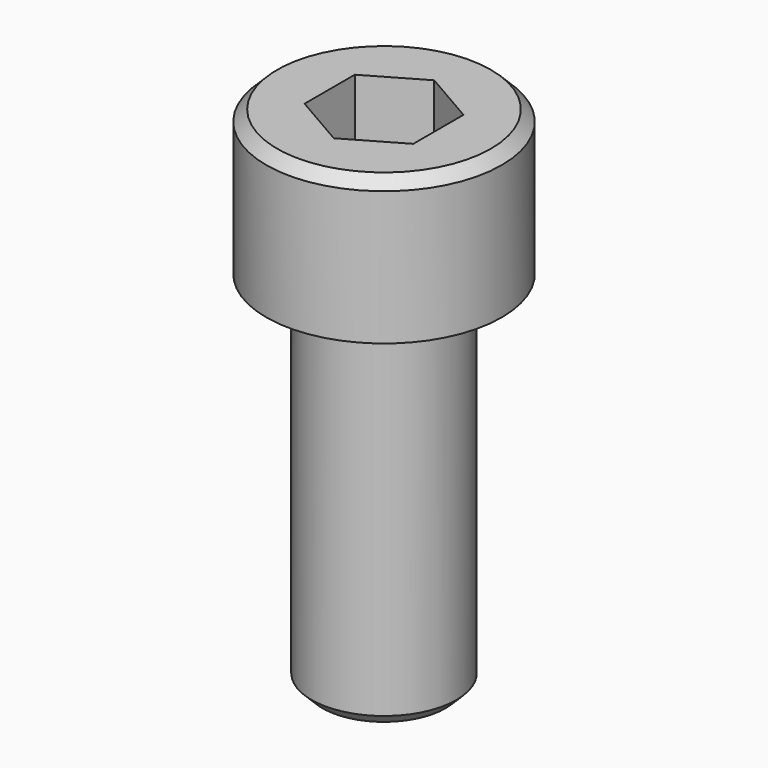
from build123d import *

# Parameters (mm, degrees)
F2_R      = 2
F3_DEPTH  = 10
F2_R_2    = 3.25
F3_FACE_R = 2
F4_DEPTH  = 4
F5_SIZE   = 0.3
F7_DEPTH  = 2


with BuildPart() as f3:
    # F2 (on Top) → F3 (new body)
    with BuildSketch(Plane.XY):
        Circle(F2_R)
    extrude(amount=-F3_DEPTH)

    # F2 (on Top) + F3_face (on face) → F4 (join)
    with BuildSketch(Plane.XY):
        Circle(F2_R_2)
        Circle(F2_R, mode=Mode.SUBTRACT)
    with BuildSketch(Plane.XY):
        Circle(F3_FACE_R)
    extrude(amount=F4_DEPTH)

    # F5
    f5_edges = [f3.edges().sort_by_distance(p)[0] for p in [
        (-2, 0, -10),
        (-3.25, 0, 4),
    ]]
    chamfer(f5_edges, length=F5_SIZE)

    # F6 (on face) → F7 (cut)
    with BuildSketch(Plane.XY.offset(4)):
        Polygon((1.5, -0.8660254038), (1.5, 0.8660254038), (0, 1.7320508076), (-1.5, 0.8660254038), (-1.5, -0.8660254038), (0, -1.7320508076), align=None)
    extrude(amount=-F7_DEPTH, mode=Mode.SUBTRACT)


solid = f3.part
